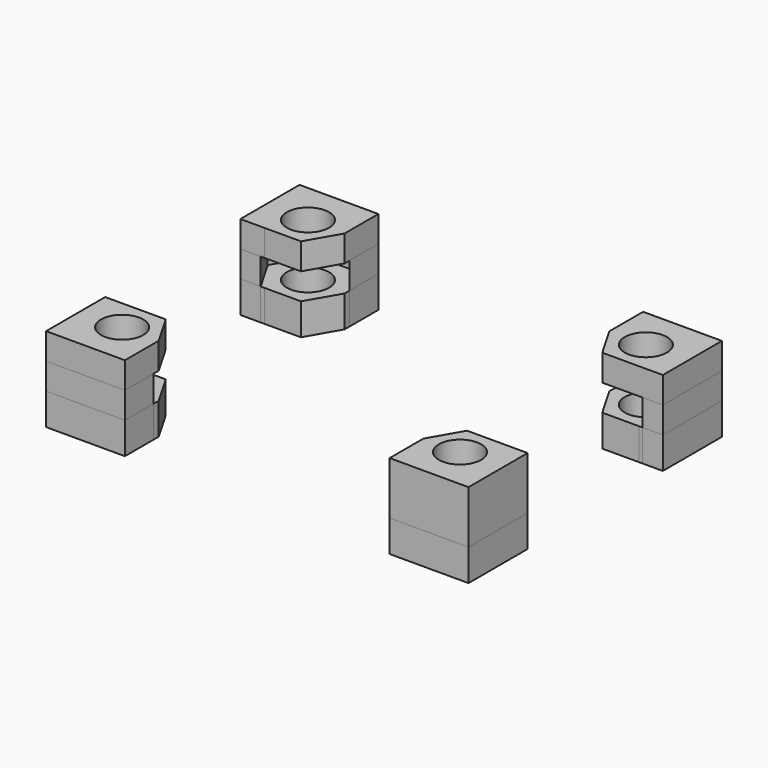
from build123d import *

# Parameters (mm, degrees)
F0_R      = 2
F1_DEPTH  = 3
F2_DEPTH  = 3
F3_DEPTH  = 2.5
F4_START  = 2.5
F1_FACE_R = 2
F4_DEPTH  = 2.5


with BuildPart() as f1:
    # F0 (on Top) → F1 (new body)
    with BuildSketch(Plane.XY):
        Polygon((56.2425711751, 29.4110085815), (56.2425711751, 36.414245103), (54.3157895307, 36.414245103), (56.0530762776, 33.4181404888), (54.1540001392, 30.1145803152), (50.3434950368, 30.1074484079), (48.7784756274, 32.8064627658), (48.7784756274, 29.4110085815), align=None)
        Polygon((56.0530762776, 33.4181404888), (54.3157895307, 36.414245103), (53.9690040281, 36.414245103), (50.5049084804, 36.4077615509), (48.7784756274, 33.4045250294), (48.7784756274, 32.8064627658), (50.3434950368, 30.1074484079), (54.1540001392, 30.1145803152), align=None)
        with Locations((52.2425711751, 33.4110085815)):
            Circle(F0_R, mode=Mode.SUBTRACT)
    extrude(amount=F1_DEPTH)


with BuildPart() as f1b:
    # F0 (on Top) → F1, piece 2 (new body)
    with BuildSketch(Plane.XY):
        Polygon((18.1588716375, 36.4077615509), (16.2425711751, 36.4077615509), (16.2425711751, 29.4110085815), (23.7066667228, 29.4110085815), (23.7066667228, 32.8155396842), (22.1540001392, 30.1145803152), (18.3434950368, 30.1074484079), (16.4320660726, 33.4038766742), align=None)
        Polygon((18.5049084804, 36.4077615509), (18.1588716375, 36.4077615509), (16.4320660726, 33.4038766742), (18.3434950368, 30.1074484079), (22.1540001392, 30.1145803152), (23.7066667228, 32.8155396842), (23.7066667228, 33.4174921336), (21.9690040281, 36.414245103), align=None)
        with Locations((20.2425711751, 33.4110085815)):
            Circle(F0_R, mode=Mode.SUBTRACT)
    extrude(amount=F1_DEPTH)


with BuildPart() as f1c:
    # F0 (on Top) → F1, piece 3 (new body)
    with BuildSketch(Plane.XY):
        Polygon((23.7066667228, 59.4110085815), (16.2425711751, 59.4110085815), (16.2425711751, 52.40777206), (18.1693528195, 52.40777206), (16.4320660726, 55.4038766742), (18.331142211, 58.7074368479), (22.1416473134, 58.7145687551), (23.7066667228, 56.0155543972), align=None)
        Polygon((23.7066667228, 55.4174921336), (23.7066667228, 56.0155543972), (22.1416473134, 58.7145687551), (18.331142211, 58.7074368479), (16.4320660726, 55.4038766742), (18.1693528195, 52.40777206), (18.5161383221, 52.40777206), (21.9802338698, 52.4142556121), align=None)
        with Locations((20.2425711751, 55.4110085815)):
            Circle(F0_R, mode=Mode.SUBTRACT)
    extrude(amount=F1_DEPTH)


with BuildPart() as f1d:
    # F0 (on Top) → F1, piece 4 (new body)
    with BuildSketch(Plane.XY):
        Polygon((56.2425711751, 59.4110085815), (48.7784756274, 59.4110085815), (48.7784756274, 56.0064774788), (50.331142211, 58.7074368479), (54.1416473134, 58.7145687551), (56.0530762776, 55.4181404888), (54.3266434245, 52.4149039673), (56.2425711751, 52.4184899011), align=None)
        Polygon((50.331142211, 58.7074368479), (48.7784756274, 56.0064774788), (48.7784756274, 55.4045250294), (50.5161383221, 52.40777206), (53.9802338698, 52.4142556121), (54.3266434245, 52.4149039673), (56.0530762776, 55.4181404888), (54.1416473134, 58.7145687551), align=None)
        with Locations((52.2425711751, 55.4110085815)):
            Circle(F0_R, mode=Mode.SUBTRACT)
    extrude(amount=F1_DEPTH)


with BuildPart() as f2:
    # F0 (on Top) → F2 (new body, through all)
    with BuildSketch(Plane.XY):
        Polygon((56.2425711751, 29.4110085815), (56.2425711751, 36.414245103), (54.3157895307, 36.414245103), (56.0530762776, 33.4181404888), (54.1540001392, 30.1145803152), (50.3434950368, 30.1074484079), (48.7784756274, 32.8064627658), (48.7784756274, 29.4110085815), align=None)
    extrude(amount=F2_DEPTH)


with BuildPart() as f2b:
    # F0 (on Top) → F2, piece 2 (new body, through all)
    with BuildSketch(Plane.XY):
        Polygon((56.2425711751, 59.4110085815), (48.7784756274, 59.4110085815), (48.7784756274, 56.0064774788), (50.331142211, 58.7074368479), (54.1416473134, 58.7145687551), (56.0530762776, 55.4181404888), (54.3266434245, 52.4149039673), (56.2425711751, 52.4184899011), align=None)
    extrude(amount=F2_DEPTH)


with BuildPart() as f2c:
    # F0 (on Top) → F2, piece 3 (new body, through all)
    with BuildSketch(Plane.XY):
        Polygon((23.7066667228, 59.4110085815), (16.2425711751, 59.4110085815), (16.2425711751, 52.40777206), (18.1693528195, 52.40777206), (16.4320660726, 55.4038766742), (18.331142211, 58.7074368479), (22.1416473134, 58.7145687551), (23.7066667228, 56.0155543972), align=None)
    extrude(amount=F2_DEPTH)


with BuildPart() as f2d:
    # F0 (on Top) → F2, piece 4 (new body, through all)
    with BuildSketch(Plane.XY):
        Polygon((18.1588716375, 36.4077615509), (16.2425711751, 36.4077615509), (16.2425711751, 29.4110085815), (23.7066667228, 29.4110085815), (23.7066667228, 32.8155396842), (22.1540001392, 30.1145803152), (18.3434950368, 30.1074484079), (16.4320660726, 33.4038766742), align=None)
    extrude(amount=F2_DEPTH)


with BuildPart() as f3:
    # F3 (new): a face of the model
    f3_faces = [f2.part.faces().sort_by_distance(p)[0] for p in [
        (52.5105234013, 29.5133599587, 3),
    ]]
    extrude(f3_faces, amount=F3_DEPTH)

    # F1_face (on face) → F4 (join)
    with BuildSketch(Plane(origin=(52.8230493213, 32.5673462874, 3), x_dir=(1, 0, 0), z_dir=(0, 0, 1)).offset(F4_START)):
        Polygon((-4.0445736939, -3.1563377059), (3.4195218538, -3.1563377059), (3.4195218538, 3.8468988156), (1.1459547068, 3.8468988156), (-2.3181408409, 3.8404152635), (-4.0445736939, 0.837178742), align=None)
        with Locations((-0.5804781462, 0.8436622941)):
            Circle(F1_FACE_R, mode=Mode.SUBTRACT)
    extrude(amount=F4_DEPTH)


with BuildPart() as f3b:
    # F3#2 (new): a face of the model
    f3_2_faces = [f2d.part.faces().sort_by_distance(p)[0] for p in [
        (17.2067727863, 34.9568067074, 3),
    ]]
    extrude(f3_2_faces, amount=F3_DEPTH)


with BuildPart() as f3c:
    # F3#3 (new): a face of the model
    f3_3_faces = [f2c.part.faces().sort_by_distance(p)[0] for p in [
        (19.9746189489, 59.3086572043, 3),
    ]]
    extrude(f3_3_faces, amount=F3_DEPTH)


with BuildPart() as f3d:
    # F3#4 (new): a face of the model
    f3_4_faces = [f2b.part.faces().sort_by_distance(p)[0] for p in [
        (52.5105234013, 59.3087059901, 3),
    ]]
    extrude(f3_4_faces, amount=F3_DEPTH)


with BuildPart() as f4:
    # F1_face (on face) → F4, piece 2 (new body)
    with BuildSketch(Plane(origin=(52.8230493213, 32.5673462874, 3), x_dir=(1, 0, 0), z_dir=(0, 0, 1)).offset(F4_START)):
        Polygon((-36.5804781462, 3.8404152635), (-36.5804781462, -3.1563377059), (-29.1163825985, -3.1563377059), (-29.1163825985, 0.8501458462), (-30.8540452932, 3.8468988156), (-34.3181408409, 3.8404152635), align=None)
        with Locations((-32.5804781462, 0.8436622941)):
            Circle(F1_FACE_R, mode=Mode.SUBTRACT)
    extrude(amount=F4_DEPTH)


with BuildPart() as f4b:
    # F1_face (on face) → F4, piece 3 (new body)
    with BuildSketch(Plane(origin=(52.8230493213, 32.5673462874, 3), x_dir=(1, 0, 0), z_dir=(0, 0, 1)).offset(F4_START)):
        Polygon((-29.1163825985, 26.8436622941), (-36.5804781462, 26.8436622941), (-36.5804781462, 19.8404257726), (-34.3069109992, 19.8404257726), (-30.8428154515, 19.8469093247), (-29.1163825985, 22.8501458462), align=None)
        with Locations((-32.5804781462, 22.8436622941)):
            Circle(F1_FACE_R, mode=Mode.SUBTRACT)
    extrude(amount=F4_DEPTH)


with BuildPart() as f4c:
    # F1_face (on face) → F4, piece 4 (new body)
    with BuildSketch(Plane(origin=(52.8230493213, 32.5673462874, 3), x_dir=(1, 0, 0), z_dir=(0, 0, 1)).offset(F4_START)):
        Polygon((3.4195218538, 26.8436622941), (-4.0445736939, 26.8436622941), (-4.0445736939, 22.837178742), (-2.3069109992, 19.8404257726), (3.4195218538, 19.8511436137), align=None)
        with Locations((-0.5804781462, 22.8436622941)):
            Circle(F1_FACE_R, mode=Mode.SUBTRACT)
    extrude(amount=F4_DEPTH)


solid = Compound([f1.part, f1b.part, f1c.part, f1d.part, f2.part, f2b.part, f2c.part, f2d.part, f3.part, f3b.part, f3c.part, f3d.part, f4.part, f4b.part, f4c.part])
